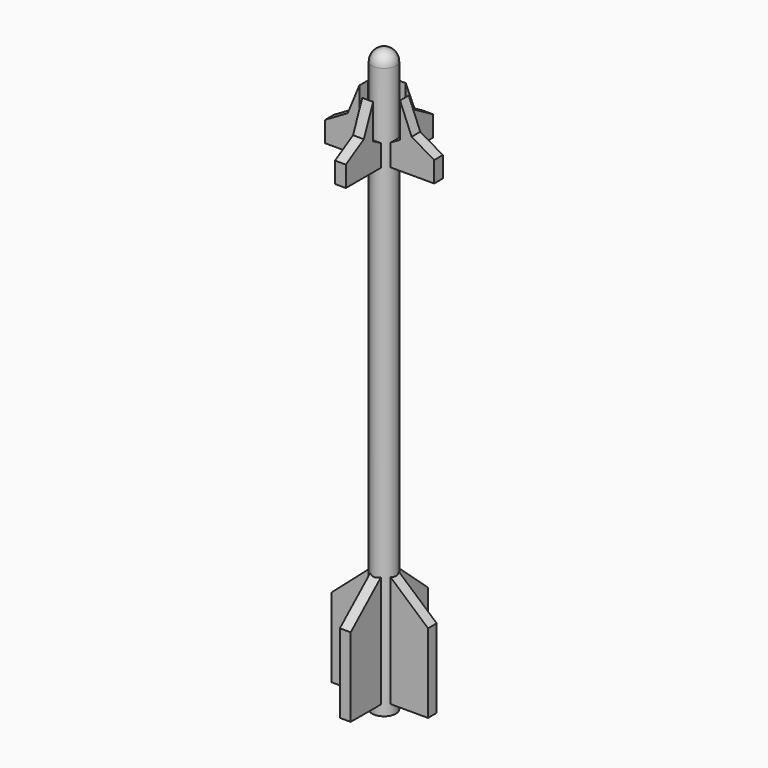
from build123d import *

# Parameters (mm, degrees)
F3_DEPTH = 0.2
F4_COUNT = 4


# Not quite as in the source:
# - a feature names something its author has since deleted; it is built from what else it names


with BuildPart() as f1:
    # F0 (on Front) → F1 (revolve)
    with BuildSketch(Plane.XZ):
        with BuildLine():
            Line((0, 21.5277777778), (0, 0))
            Line((0, 0), (0.4409722222, 0))
            Line((0.4409722222, 0), (0.4409722222, 21.0868055556))
            ThreePointArc((0.4409722222, 21.0868055556), (0.3118144486, 21.3986200042), (0, 21.5277777778))
        make_face()
    revolve(axis=Axis((0, 0, 10.7638888889), (0, 0, 1)))

    # F2 (on Front) → F3 (join, symmetric)
    with BuildSketch(Plane.XZ):
        Polygon((0, 18.4355709877), (0, 17.8472222222), (2.0138888889, 17.8472222222), (2.0138888889, 18.6111111111), (1.1805555556, 19.0972222222), (0.7534722222, 20.1388888889), (0.7534722222, 18.8541666667), align=None)
        Polygon((0, 4.8655856243), (0, 0.3819444444), (1.7881944444, 0.3819444444), (1.7881944444, 3.2986111111), align=None)
    extrude(amount=F3_DEPTH, both=True)

    # F4: F1 ×4 about axis
    f4_axis = Axis((0, 0, 0), (0, 0, 1))


with BuildPart() as f1_1:
    add(f1.part)
    for i in range(1, F4_COUNT):
        add(f1.part.rotate(f4_axis, i * 360 / F4_COUNT))


solid = f1_1.part
